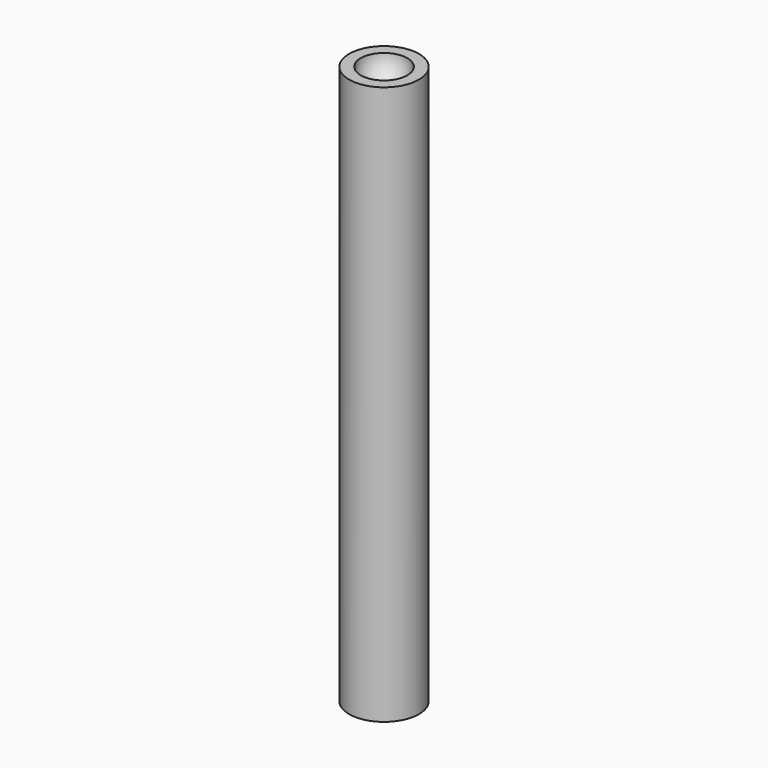
from build123d import *

# Parameters (mm, degrees)
F0_R     = 4.7625
F1_DEPTH = 76.2
F2_R     = 3.175
F3_DEPTH = 3.175
F4_R     = 3.17499
F5_R     = 3.175
F6_DEPTH = 69.85
F7_R     = 3.175


# Not quite as in the source:
# - a fillet or chamfer is up to 0.001 mm smaller than in the source, because OpenCascade refuses the exact size


with BuildPart() as f1:
    # F0 (on Top) → F1 (new body)
    with BuildSketch(Plane.XY):
        Circle(F0_R)
    extrude(amount=F1_DEPTH)

    # F2 (on face) → F3 (cut)
    with BuildSketch(Plane.XY.offset(76.2)):
        Circle(F2_R)
    extrude(amount=-F3_DEPTH, mode=Mode.SUBTRACT)

    # F4 (radius 3.175 in the source; OpenCascade refuses exactly that, so slightly less here)
    f4_edges = [f1.edges().sort_by_distance(p)[0] for p in [
        (-3.175, 0, 73.025),
    ]]
    fillet(f4_edges, radius=F4_R)

    # F5 (on face) → F6 (cut)
    with BuildSketch(Plane(origin=(0, 0, 0), x_dir=(1, 0, 0), z_dir=(0, 0, -1))):
        Circle(F5_R)
    extrude(amount=-F6_DEPTH, mode=Mode.SUBTRACT)

    # F7
    f7_edges = [f1.edges().sort_by_distance(p)[0] for p in [
        (-3.175, 0, 69.85),
    ]]
    fillet(f7_edges, radius=F7_R)


solid = f1.part
